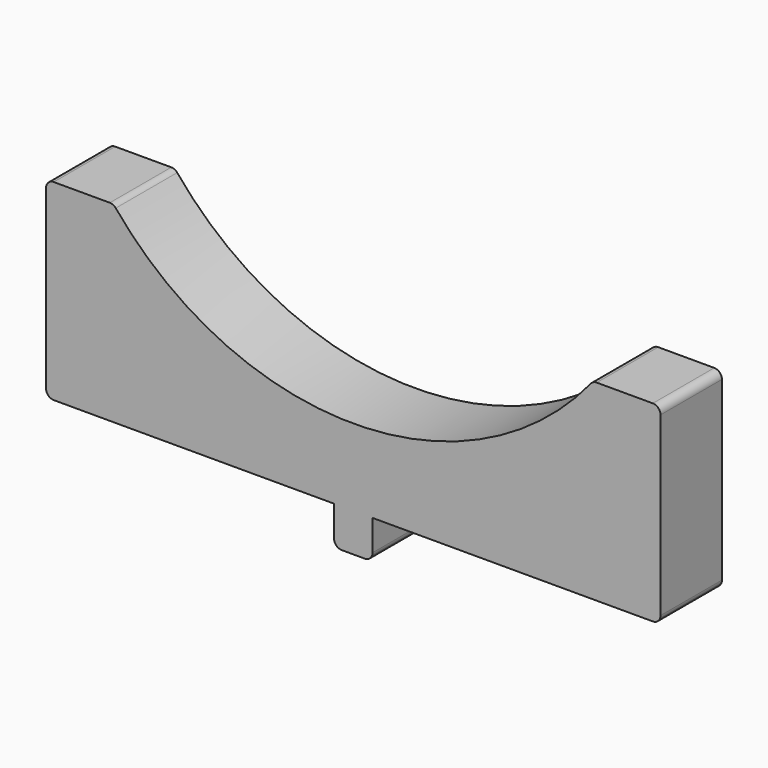
from build123d import *

# Parameters (mm, degrees)
F0_W     = 101.6
F0_H     = 31.75
F1_DEPTH = 6.35
F3_DEPTH = 12.7
F4_W     = 6.35
F4_H     = 12.7
F5_DEPTH = 6.35
F6_R     = 1.27


with BuildPart() as f1:
    # F0 (on Front) → F1 (new body, symmetric)
    with BuildSketch(Plane.XZ):
        Rectangle(F0_W, F0_H)
    extrude(amount=F1_DEPTH, both=True)

    # F2 (on Front) → F3 (cut, symmetric)
    with BuildSketch(Plane.XZ):
        with BuildLine():
            Line((39.6557372898, 15.875), (-39.6557372898, 15.875))
            ThreePointArc((-39.6557372898, 15.875), (0, -3.175), (39.6557372898, 15.875))
        make_face()
    extrude(amount=F3_DEPTH, both=True, mode=Mode.SUBTRACT)

    # F4 (on face) → F5 (join)
    with BuildSketch(Plane(origin=(0, 0, -15.875), x_dir=(1, 0, 0), z_dir=(0, 0, -1))):
        Rectangle(F4_W, F4_H)
    extrude(amount=F5_DEPTH)

    # F6
    f6_edges = [f1.edges().sort_by_distance(p)[0] for p in [
        (-3.175, 0, -22.225),
        (3.175, 0, -22.225),
        (-50.8, 0, -15.875),
        (-50.8, 0, 15.875),
        (-39.655737, 0, 15.875),
        (39.655737, 0, 15.875),
        (50.8, 0, 15.875),
        (50.8, 0, -15.875),
    ]]
    fillet(f6_edges, radius=F6_R)


solid = f1.part
